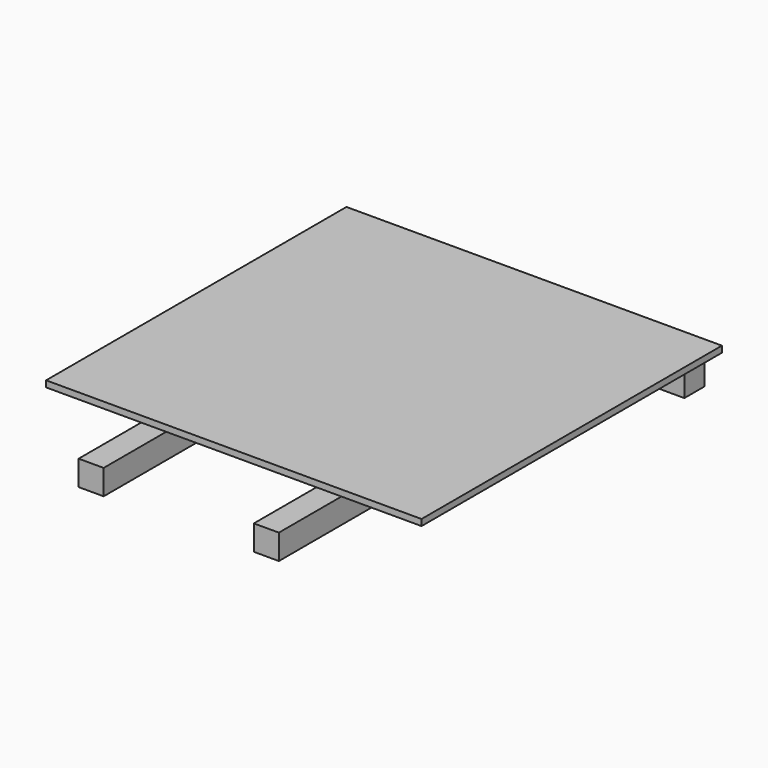
from build123d import *

# Parameters (mm, degrees)
F1_START = 25
F0_W     = 20
F0_H     = 275
F0_W_2   = 120
F0_W_3   = 60
F0_H_2   = 20
F1_DEPTH = 5
F0_H_3   = 55
F2_DEPTH = 20


# Not quite as in the source:
# - a feature names something its author has since deleted; it is built from what else it names


with BuildPart() as f1:
    # F0 (on Top) → F1 (new body)
    with BuildSketch(Plane.XY.offset(F1_START)):
        Polygon((150, -150), (150, 150), (-150, 150), (-150, -150), (-80, -150), (-80, 125), (-140, 125), (-140, 145), (-80, 145), (-60, 145), (60, 145), (80, 145), (140, 145), (140, 125), (80, 125), (80, -150), align=None)
        with Locations((-70, -12.5)):
            Rectangle(F0_W, F0_H)
        with Locations((0, -12.5)):
            Rectangle(F0_W_2, F0_H)
        with Locations((70, -12.5)):
            Rectangle(F0_W, F0_H)
        with Locations((-110, 135)):
            Rectangle(F0_W_3, F0_H_2)
        with Locations((-70, 135)):
            Rectangle(F0_W, F0_H_2)
        with Locations((0, 135)):
            Rectangle(F0_W_2, F0_H_2)
        with Locations((70, 135)):
            Rectangle(F0_W, F0_H_2)
        with Locations((110, 135)):
            Rectangle(F0_W_3, F0_H_2)
    extrude(amount=F1_DEPTH)


with BuildPart() as f2:
    # F0 (on Top) → F2 (new body)
    with BuildSketch(Plane.XY):
        with Locations((-110, 135)):
            Rectangle(F0_W_3, F0_H_2)
        with Locations((-70, 135)):
            Rectangle(F0_W, F0_H_2)
        with Locations((0, 135)):
            Rectangle(F0_W_2, F0_H_2)
        with Locations((70, 135)):
            Rectangle(F0_W, F0_H_2)
        with Locations((110, 135)):
            Rectangle(F0_W_3, F0_H_2)
        with Locations((70, -12.5)):
            Rectangle(F0_W, F0_H)
        with Locations((-70, -12.5)):
            Rectangle(F0_W, F0_H)
        with Locations((-70, -177.5)):
            Rectangle(F0_W, F0_H_3)
        with Locations((70, -177.5)):
            Rectangle(F0_W, F0_H_3)
    extrude(amount=F2_DEPTH)


solid = Compound([f1.part, f2.part])
